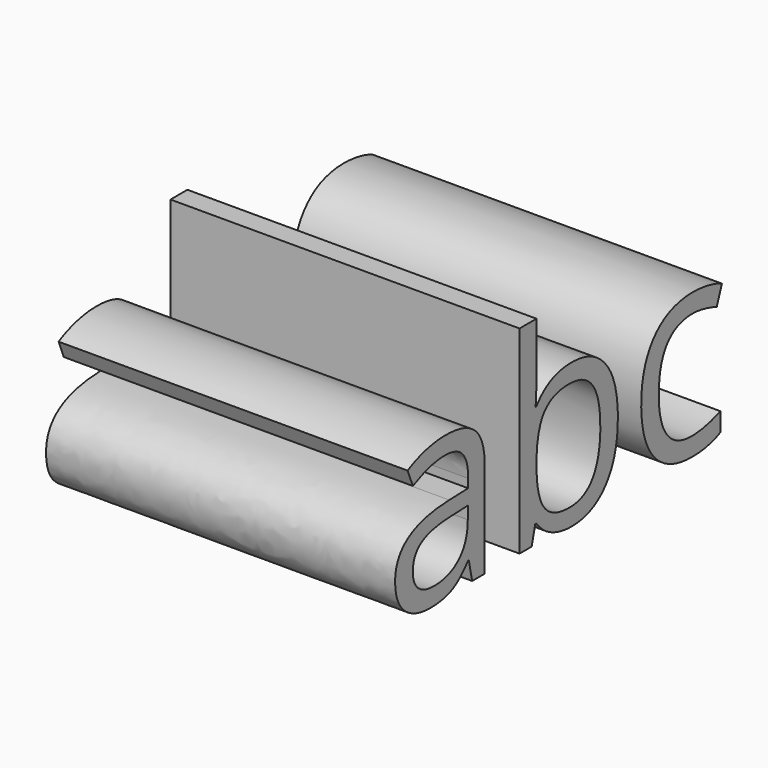
from build123d import *

# Parameters (mm, degrees)
F0_TEXT_SIZE = 57.5230004162
F1_DEPTH     = 76.962


# Not quite as in the source:
# - Text() gives the source's letters only with a copy of the font that has no kerning and outlines rounded to 1/6400 em; it was checked with that copy


with BuildPart() as f1:
    # F0 (on Right) → F1 (new body)
    with BuildSketch(Plane.YZ):
        with Locations((-35.4461744428, -28.9518050849)):
            Text('abc', F0_TEXT_SIZE, font='Open Sans', text_align=(TextAlign.LEFT, TextAlign.BOTTOM))
    extrude(amount=F1_DEPTH)


solid = f1.part
